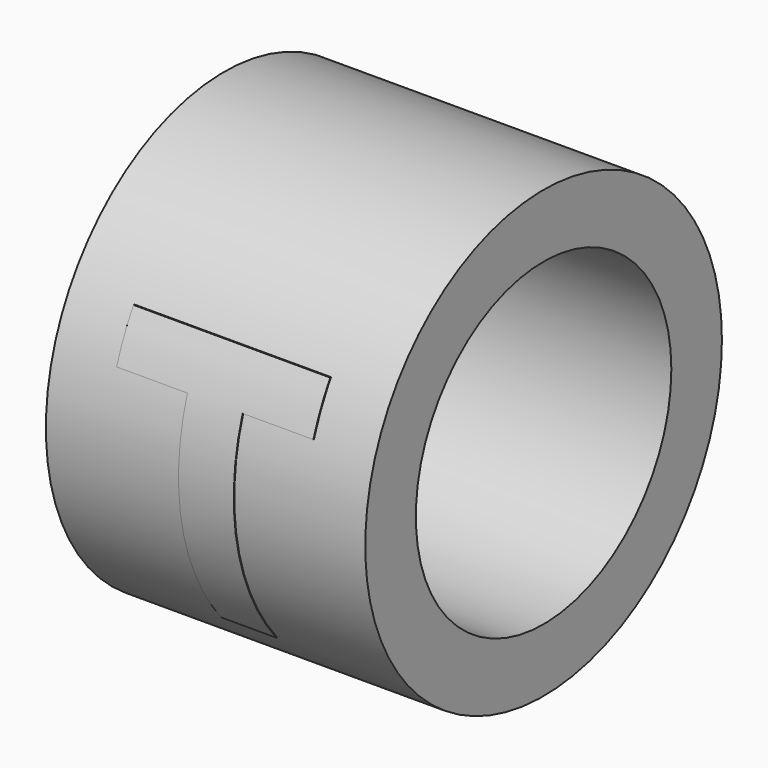
from build123d import *

# Parameters (mm, degrees)
F0_R         = 1.75
F0_R_2       = 1.745
F0_R_3       = 1.25
F1_DEPTH     = 2.5
F2_TEXT_SIZE = 2.8570699214
F3_REACH     = 4.3068410995
F4_DEPTH     = 2.5


# Not quite as in the source:
# - Text() gives the source's letters only with a copy of the font that has no kerning and outlines rounded to 1/6400 em; it was checked with that copy


with BuildPart() as f1:
    # F0 (on Right) → F1 (new body)
    with BuildSketch(Plane.YZ):
        Circle(F0_R)
        Circle(F0_R_2, mode=Mode.SUBTRACT)
        Circle(F0_R_2)
        Circle(F0_R_3, mode=Mode.SUBTRACT)
    extrude(amount=F1_DEPTH)

    f3_end = f1.faces().sort_by_distance((1.25, -1.75, 0))[0]
    # F2 (on Front) → F3 (intersect, up to a face of the model that its end follows)
    with BuildSketch(Plane.XZ):
        with Locations((0.4309935612, -1.1343103251)):
            Text('T', F2_TEXT_SIZE, font='Open Sans', font_style=FontStyle.BOLD, text_align=(TextAlign.LEFT, TextAlign.BOTTOM))
    f3_long = extrude(amount=F3_REACH, mode=Mode.PRIVATE)
    add(split(f3_long, bisect_by=f3_end, keep=Keep.BOTTOM, mode=Mode.PRIVATE), mode=Mode.INTERSECT)


with BuildPart() as f4:
    # F0 (on Right) → F4 (new body)
    with BuildSketch(Plane.YZ):
        Circle(F0_R_2)
        Circle(F0_R_3, mode=Mode.SUBTRACT)
    extrude(amount=F4_DEPTH)


solid = Compound([f1.part, f4.part])
